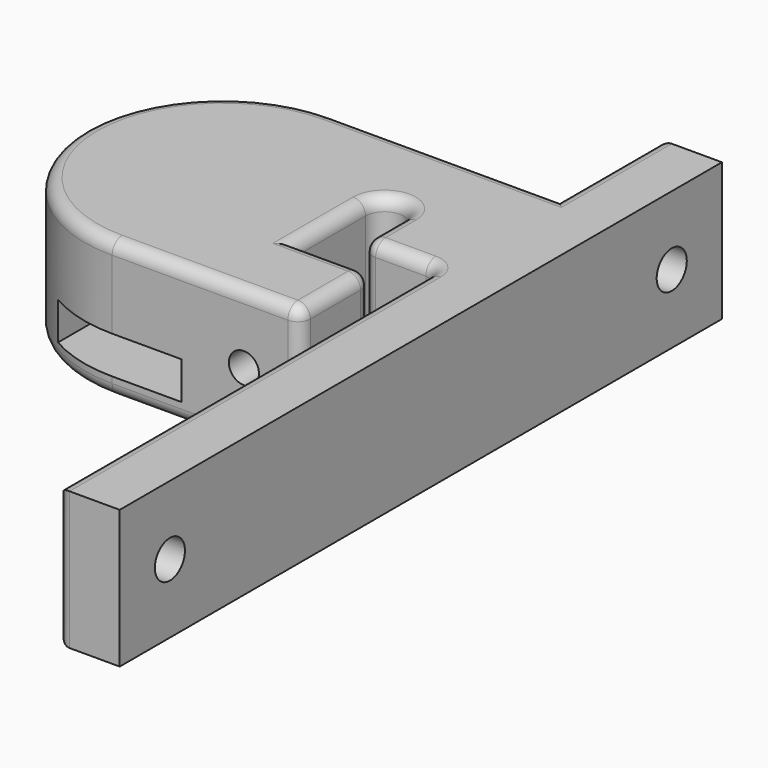
from build123d import *

# Parameters (mm, degrees)
F1_DEPTH  = 5.5
F2_R      = 1.5
F3_DEPTH  = 25
F5_START  = -0.5
F4_R      = 5.5
F5_DEPTH  = 9
F7_START  = -1.5
F6_W      = 11
F6_H      = 16.464828267
F7_DEPTH  = 3
F8_R      = 1
F9_DEPTH  = 25
F11_DEPTH = 25
F12_R     = 1.2
F13_DEPTH = 7
F14_R     = 1


with BuildPart() as f1:
    # F0 (on Top) → F1 (new body, symmetric)
    with BuildSketch(Plane.XY):
        with BuildLine():
            Line((18, 11), (0, 11))
            ThreePointArc((0, 11), (-11, 0), (0, -11))
            Line((0, -11), (18, -11))
            Line((18, -11), (18, -39))
            Line((18, -39), (23, -39))
            Line((23, -39), (23, 21))
            Line((23, 21), (18, 21))
            Line((18, 21), (18, 11))
        make_face()
    extrude(amount=F1_DEPTH, both=True)

    # F2 (on face) → F3 (cut)
    with BuildSketch(Plane.YZ.offset(23)):
        with Locations((16, 0)):
            Circle(F2_R)
        with Locations((-34, 0)):
            Circle(F2_R)
    extrude(amount=-F3_DEPTH, mode=Mode.SUBTRACT)

    # F4 (on face) → F5 (cut)
    with BuildSketch(Plane.XY.offset(5.5).offset(F5_START)):
        Circle(F4_R)
    extrude(amount=-F5_DEPTH, mode=Mode.SUBTRACT)

    # F6 (on face) → F7 (cut)
    with BuildSketch(Plane(origin=(0, 0, -5.5), x_dir=(1, 0, 0), z_dir=(0, 0, -1)).offset(F7_START)):
        with Locations((0.0076012546, 8.2324141335)):
            Rectangle(F6_W, F6_H)
    extrude(amount=-F7_DEPTH, mode=Mode.SUBTRACT)

    # F8 (on face) → F9 (cut)
    with BuildSketch(Plane.XZ.offset(11)):
        with Locations((0, -2.5)):
            Circle(F8_R)
    extrude(amount=-F9_DEPTH, mode=Mode.SUBTRACT)

    # F10 (on face) → F11 (cut)
    with BuildSketch(Plane.XY.offset(5.5)):
        with BuildLine():
            Line((12, -1), (12, 3))
            ThreePointArc((12, 3), (10.5, 4.5), (9, 3))
            Line((9, 3), (9, -4))
            Line((9, -4), (15, -4))
            Line((15, -4), (15, -11))
            Line((15, -11), (18, -11))
            Line((18, -11), (18, -1))
            Line((18, -1), (12, -1))
        make_face()
    extrude(amount=-F11_DEPTH, mode=Mode.SUBTRACT)

    # F12 (on face) → F13 (cut, through all)
    with BuildSketch(Plane.XZ.offset(11)):
        with Locations((10.5, 0)):
            Circle(F12_R)
    extrude(amount=-F13_DEPTH, mode=Mode.SUBTRACT)

    # F14
    f14_edges = [f1.edges().sort_by_distance(p)[0] for p in [
        (18, 16, 5.5),
        (18, 21, 0),
        (18, 16, -5.5),
        (9, 11, 5.5),
        (18, -20, 5.5),
        (-11, 0, -5.5),
        (7.5, -11, -5.5),
        (18, -20, -5.5),
        (15, -1, -5.5),
        (18, -39, 0),
        (18, -1, 0),
        (12, 1, 5.5),
        (12, -4, 5.5),
        (15, -7.5, -5.5),
        (15, -7.5, 5.5),
        (15, -11, 0),
        (15, -4, 0),
        (12, -1, 0),
        (9, -0.5, -5.5),
        (12, -4, -5.5),
        (9, 11, -5.5),
        (-11, 0, 5.5),
        (7.5, -11, 5.5),
        (9, -0.5, 5.5),
        (10.5, 4.5, 5.5),
        (15, -1, 5.5),
        (10.5, 4.5, -5.5),
    ]]
    fillet(f14_edges, radius=F14_R)


solid = f1.part
